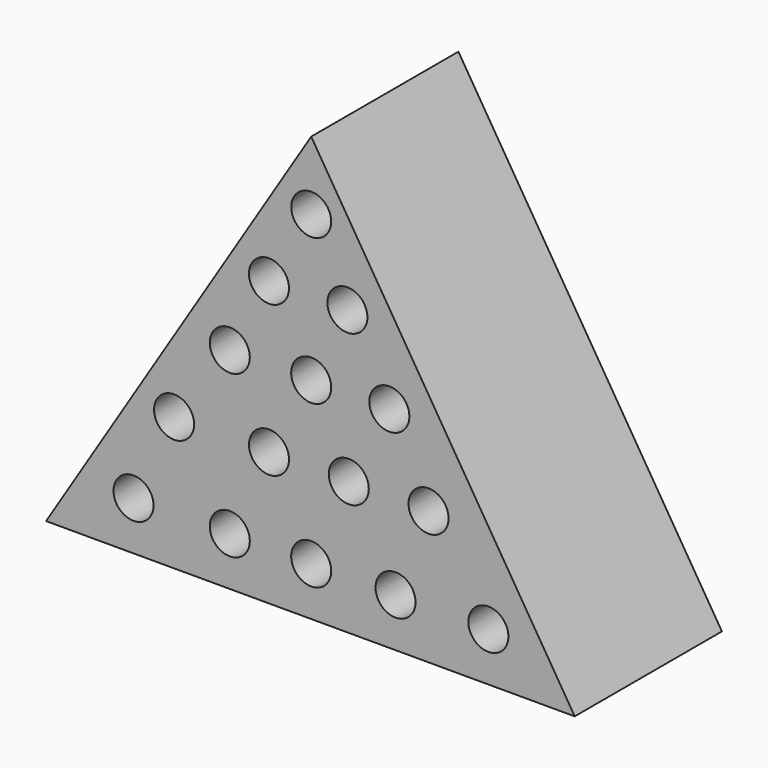
from build123d import *

# Parameters (mm, degrees)
F1_DEPTH = 1.016
F2_DEPTH = 17.78
F3_R     = 2.0447
F3_R_2   = 2.0406784107
F4_DEPTH = 12.7


# Not quite as in the source:
# - a feature names something its author has since deleted; it is built from what else it names


with BuildPart() as f1:
    # F0 (on Front) → F1 (new body)
    with BuildSketch(Plane.XZ):
        Polygon((-27.083877352, 12.2783370181), (26.9169844677, 12.2783370181), (0, 55.663280189), align=None)
    extrude(amount=F1_DEPTH)

    # F2 (add): a face of the model
    f2_faces = [f1.faces().sort_by_distance(p)[0] for p in [
        (-0.0556309614, -1.016, 26.7399847417),
    ]]
    extrude(f2_faces, amount=F2_DEPTH)

    # F3 (on face) → F4 (cut)
    with BuildSketch(Plane.XZ.offset(18.796)):
        with Locations((3.6953620147, 41.2761941552)):
            Circle(F3_R)
        with Locations((0, 48.6748889089)):
            Circle(F3_R_2)
        with Locations((-4.3132207356, 41.2761941552)):
            Circle(F3_R)
        with Locations((0, 33.7593667209)):
            Circle(F3_R)
        with Locations((7.9806558788, 33.7593667209)):
            Circle(F3_R)
        with Locations((-8.3175115287, 33.7593667209)):
            Circle(F3_R)
        with Locations((-4.3132207356, 25.8912853897)):
            Circle(F3_R)
        with Locations((-14.0078207478, 25.8912853897)):
            Circle(F3_R)
        with Locations((3.8358634338, 25.8912853897)):
            Circle(F3_R)
        with Locations((11.9849471375, 25.8912853897)):
            Circle(F3_R)
        with Locations((18.096761778, 17.2504447401)):
            Circle(F3_R)
        with Locations((8.6129121482, 17.2504447401)):
            Circle(F3_R)
        with Locations((0, 17.2504447401)):
            Circle(F3_R)
        with Locations((-8.3175115287, 17.2504447401)):
            Circle(F3_R)
        with Locations((-18.1526131928, 17.2504447401)):
            Circle(F3_R)
    extrude(amount=-F4_DEPTH, mode=Mode.SUBTRACT)


solid = f1.part
